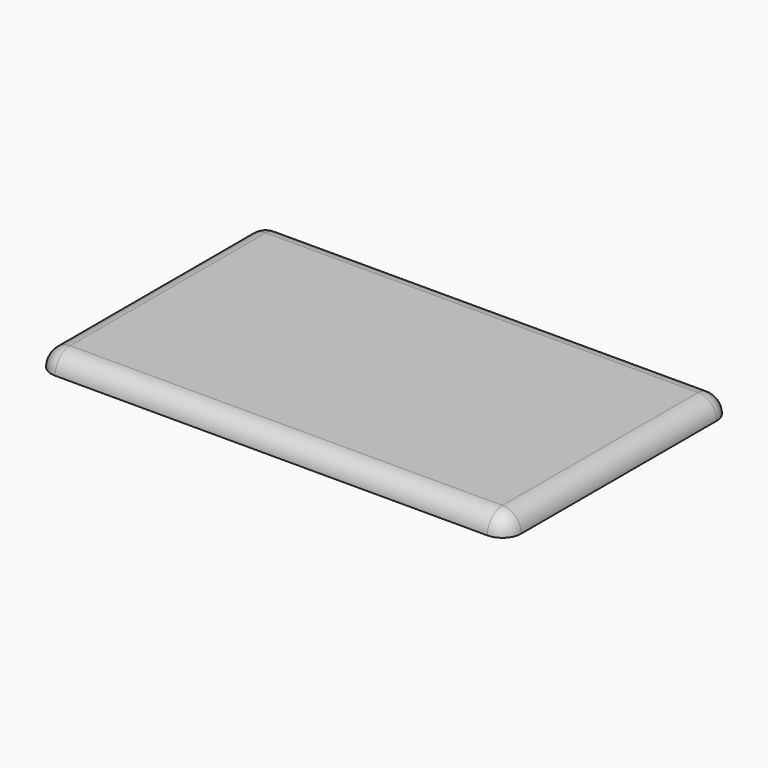
from build123d import *

# Parameters (mm, degrees)
F1_DEPTH = 5.08
F2_R     = 5.07999


# Not quite as in the source:
# - a fillet or chamfer is up to 0.001 mm smaller than in the source, because OpenCascade refuses the exact size


with BuildPart() as f1:
    # F0 (on Top) → F1 (new body)
    with BuildSketch(Plane.XY):
        with BuildLine():
            Line((121.92, 76.2), (5.08, 76.2))
            ThreePointArc((5.08, 76.2), (1.4878975516, 74.7121024484), (0, 71.12))
            Line((0, 71.12), (0, 5.08))
            ThreePointArc((0, 5.08), (1.4878975516, 1.4878975516), (5.08, 0))
            Line((5.08, 0), (121.92, 0))
            ThreePointArc((121.92, 0), (125.5121024484, 1.4878975516), (127, 5.08))
            Line((127, 5.08), (127, 71.12))
            ThreePointArc((127, 71.12), (125.5121024484, 74.7121024484), (121.92, 76.2))
        make_face()
    extrude(amount=F1_DEPTH)

    # F2 (radius 5.08 in the source; OpenCascade refuses exactly that, so slightly less here)
    f2_edges = [f1.edges().sort_by_distance(p)[0] for p in [
        (63.5, 76.2, 5.08),
        (1.487898, 74.712102, 5.08),
        (0, 38.1, 5.08),
        (1.487898, 1.487898, 5.08),
        (63.5, 0, 5.08),
        (125.512102, 1.487898, 5.08),
        (127, 38.1, 5.08),
        (125.512102, 74.712102, 5.08),
    ]]
    fillet(f2_edges, radius=F2_R)


solid = f1.part
